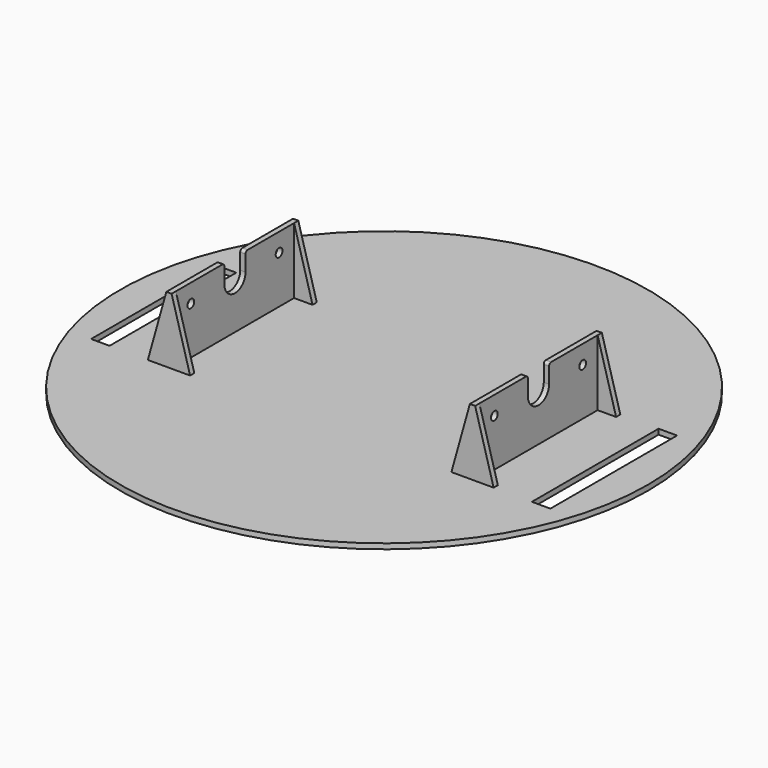
from build123d import *

# Parameters (mm, degrees)
F0_R       = 100
F0_W       = 7
F0_H       = 60
F1_DEPTH   = 2
F2_W       = 7
F2_H       = 2
F2_W_2     = 2
F2_H_2     = 56
F3_DEPTH   = 25
F4_SIZE2   = 6.99999
F4_SIZE    = 24.99999
F4_2_SIZE2 = 6.99999
F4_2_SIZE  = 24.99999
F4_3_SIZE2 = 6.99999
F4_3_SIZE  = 24.99999
F4_4_SIZE2 = 6.99999
F4_4_SIZE  = 24.99999
F5_R       = 1.6
F6_DEPTH   = 2
F7_R       = 1
F8_COUNT   = 2


# Not quite as in the source:
# - a fillet or chamfer is up to 0.001 mm smaller than in the source, because OpenCascade refuses the exact size
# - a feature names something its author has since deleted; it is built from what else it names


with BuildPart() as f1:
    # F0 (on Top) → F1 (new body)
    with BuildSketch(Plane.XY):
        Circle(F0_R)
        with Locations((-83.5, 0)):
            Rectangle(F0_W, F0_H, mode=Mode.SUBTRACT)
        with Locations((83.5, 0)):
            Rectangle(F0_W, F0_H, mode=Mode.SUBTRACT)
    extrude(amount=F1_DEPTH)


with BuildPart() as f3:
    # F2 (on face) → F3 (new body)
    with BuildSketch(Plane.XY.offset(2)):
        with Locations((-62, 29)):
            Rectangle(F2_W, F2_H)
        with Locations((-57.5, 29)):
            Rectangle(F2_W_2, F2_H)
        with Locations((-53, 29)):
            Rectangle(F2_W, F2_H)
        with Locations((-57.5, 0)):
            Rectangle(F2_W_2, F2_H_2)
        with Locations((-57.5, -29)):
            Rectangle(F2_W_2, F2_H)
        with Locations((-62, -29)):
            Rectangle(F2_W, F2_H)
        with Locations((-53, -29)):
            Rectangle(F2_W, F2_H)
    extrude(amount=F3_DEPTH)

    # F4 (size 25 and 7 in the source; OpenCascade refuses exactly that, so slightly less here)
    f4_edges = [f3.edges().sort_by_distance(p)[0] for p in [
        (-65.5, 29, 27),
    ]]
    f4_side = f3.faces().sort_by_distance((-65.5, 29, 14.5))[0]
    chamfer(f4_edges, length=F4_SIZE, length2=F4_SIZE2, reference=f4_side)

    # F4#2 (size 25 and 7 in the source; OpenCascade refuses exactly that, so slightly less here)
    f4_2_edges = [f3.edges().sort_by_distance(p)[0] for p in [
        (-49.5, 29, 27),
    ]]
    f4_2_side = f3.faces().sort_by_distance((-49.5, 29, 14.5))[0]
    chamfer(f4_2_edges, length=F4_2_SIZE, length2=F4_2_SIZE2, reference=f4_2_side)

    # F4#3 (size 25 and 7 in the source; OpenCascade refuses exactly that, so slightly less here)
    f4_3_edges = [f3.edges().sort_by_distance(p)[0] for p in [
        (-65.5, -29, 27),
    ]]
    f4_3_side = f3.faces().sort_by_distance((-65.5, -29, 14.5))[0]
    chamfer(f4_3_edges, length=F4_3_SIZE, length2=F4_3_SIZE2, reference=f4_3_side)

    # F4#4 (size 25 and 7 in the source; OpenCascade refuses exactly that, so slightly less here)
    f4_4_edges = [f3.edges().sort_by_distance(p)[0] for p in [
        (-49.5, -29, 27),
    ]]
    f4_4_side = f3.faces().sort_by_distance((-49.5, -29, 14.5))[0]
    chamfer(f4_4_edges, length=F4_4_SIZE, length2=F4_4_SIZE2, reference=f4_4_side)

    # F5 (on face) → F6 (cut)
    with BuildSketch(Plane(origin=(-58.5, 0, 0), x_dir=(0, -1, 0), z_dir=(-1, 0, 0))):
        with Locations((-20.9, 20)):
            Circle(F5_R)
        with Locations((20.9, 20)):
            Circle(F5_R)
        with BuildLine():
            ThreePointArc((-5, 20), (0, 15), (5, 20))
            ThreePointArc((5, 20), (0, 25), (-5, 20))
        make_face()
        with BuildLine():
            ThreePointArc((-5, 20), (0, 25), (5, 20))
            Line((5, 20), (5, 27))
            Line((5, 27), (-5, 27))
            Line((-5, 27), (-5, 20))
        make_face()
    extrude(amount=-F6_DEPTH, mode=Mode.SUBTRACT)

    # F7
    f7_edges = [f3.edges().sort_by_distance(p)[0] for p in [
        (-57.5, 5, 27),
        (-57.5, -5, 27),
    ]]
    fillet(f7_edges, radius=F7_R)


with BuildPart() as f8_1:
    # F8: instance of F3
    add(f3.part.rotate(Axis((0, 0, 2), (0, 0, 1)), 1 * 360 / F8_COUNT))


solid = Compound([f1.part, f3.part, f8_1.part])
